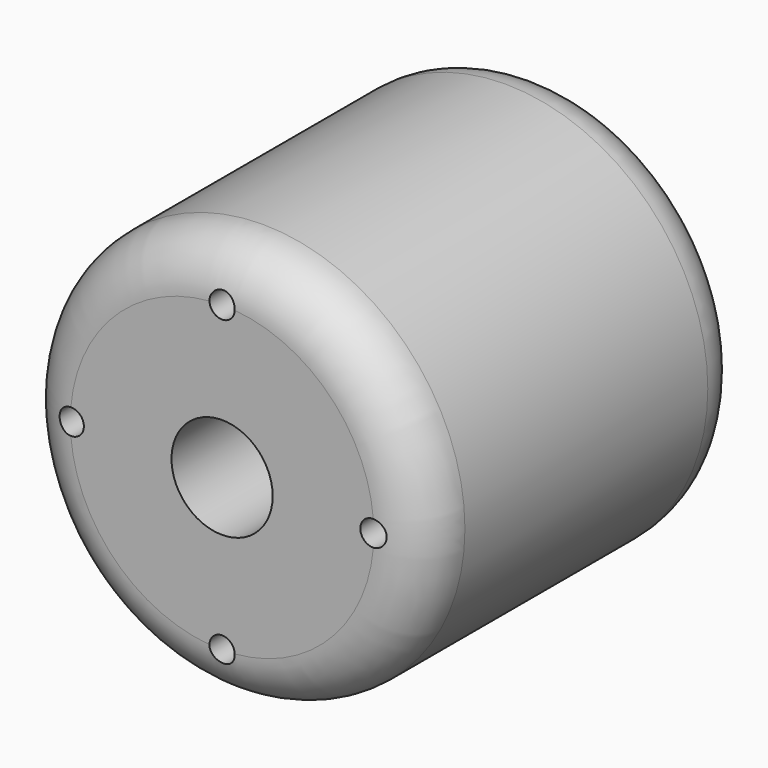
from build123d import *

# Parameters (mm, degrees)
F0_R     = 25.4
F1_DEPTH = 50.8
F2_R     = 6.35
F3_DEPTH = 50.8
F4_R     = 1.5875
F5_DEPTH = 44.45
F7_R     = 6.35


# Not quite as in the source:
# - a fillet or chamfer that OpenCascade refuses, or shapes differently, is made with other operations: its cross-section is extruded or revolved along the edge and cut away or added


with BuildPart() as f1:
    # F0 (on Front) → F1 (new body)
    with BuildSketch(Plane.XZ):
        Circle(F0_R)
    extrude(amount=F1_DEPTH)

    # F2 (on face) → F3 (cut)
    with BuildSketch(Plane.XZ.offset(50.8)):
        Circle(F2_R)
    extrude(amount=-F3_DEPTH, mode=Mode.SUBTRACT)

    # F4 (on face) → F5 (cut)
    with BuildSketch(Plane.XZ.offset(50.8)):
        with Locations((0, 19.0319661051)):
            Circle(F4_R)
        with Locations((18.9372766763, 0)):
            Circle(F4_R)
        with Locations((0, -19.0319661051)):
            Circle(F4_R)
        with Locations((-18.9372785389, 0)):
            Circle(F4_R)
    extrude(amount=-F5_DEPTH, mode=Mode.SUBTRACT)

    # F6: fillet of radius 6.35 on 1 edges, made by hand

    # F6_s1 → F6_t2 (revolve, cut)
    with BuildSketch(Plane.XY):
        with BuildLine():
            ThreePointArc((25.4, -44.45), (23.5401280605, -48.9401280605), (19.05, -50.8))
            Line((19.05, -50.8), (25.4, -50.8))
            Line((25.4, -50.8), (25.4, -44.45))
        make_face()
    revolve(axis=Axis((0, -50.8, 0), (0, -1, 0)), mode=Mode.SUBTRACT)

    # F7
    f7_edges = [f1.edges().sort_by_distance(p)[0] for p in [
        (-25.4, 0, 0),
    ]]
    fillet(f7_edges, radius=F7_R)


solid = f1.part
